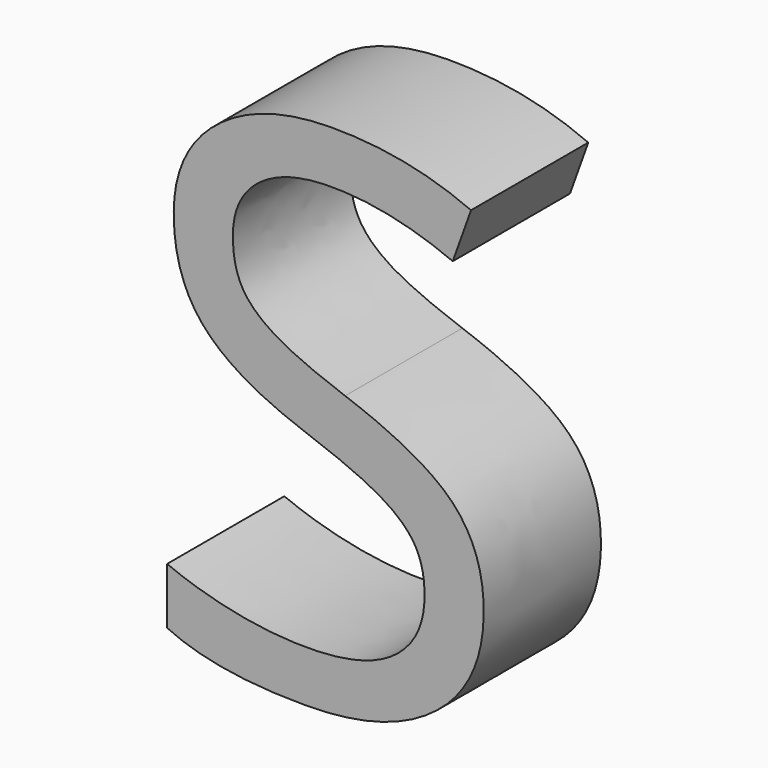
from build123d import *

# Parameters (mm, degrees)
F0_TEXT_SIZE = 120.2341376079
F1_DEPTH     = 25


# Not quite as in the source:
# - Text() gives the source's letters only with a copy of the font that has no kerning and outlines rounded to 1/6400 em; it was checked with that copy


with BuildPart() as f1:
    # F0 (on Front) → F1 (new body)
    with BuildSketch(Plane.XZ):
        with Locations((-35.868730396, -48.4446175396)):
            Text('S', F0_TEXT_SIZE, font='Open Sans', text_align=(TextAlign.LEFT, TextAlign.BOTTOM))
    extrude(amount=F1_DEPTH)


solid = f1.part
